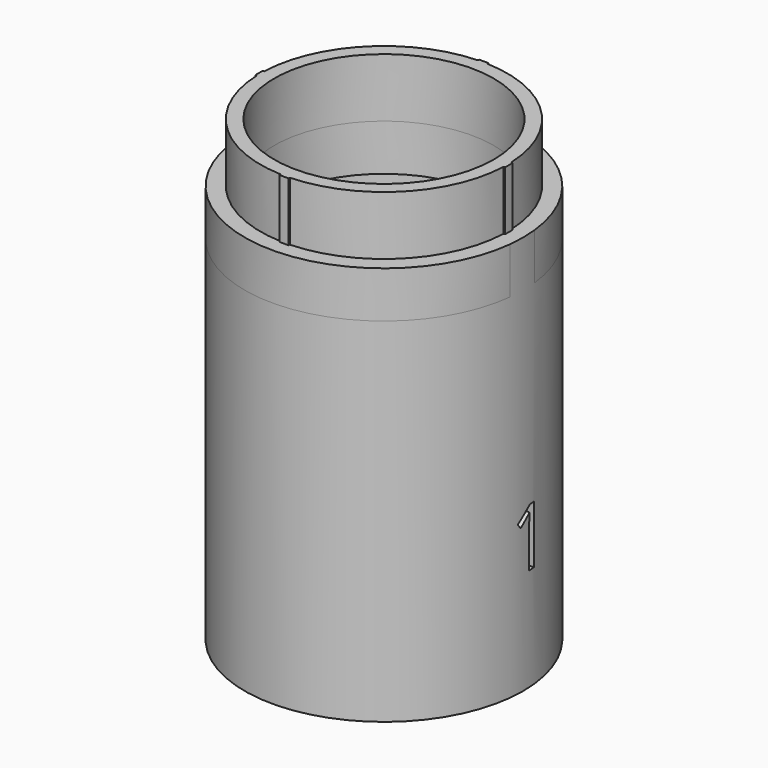
from build123d import *

# Parameters (mm, degrees)
F0_R         = 11.825
F1_DEPTH     = 6.35
F2_R         = 15
F2_R_2       = 13.45
F3_DEPTH     = 43
F4_R         = 15
F4_R_2       = 11.825
F5_DEPTH     = 5
F6_TEXT_SIZE = 8.7370552743
F7_DEPTH     = 25


# Not quite as in the source:
# - Text() gives the source's letters only with a copy of the font that has no kerning and outlines rounded to 1/6400 em; it was checked with that copy


with BuildPart() as f1:
    # F0 (on Top) → F1 (new body)
    with BuildSketch(Plane.XY):
        with BuildLine():
            ThreePointArc((13.2905981807, -0.5), (13.2976493374, -0.2500441932), (13.3, 0))
            ThreePointArc((13.3, 0), (13.2976493374, 0.2500441932), (13.2905981807, 0.5))
            ThreePointArc((13.2905981807, 0.5), (9.4045201898, 9.4045201898), (0.5, 13.2905981807))
            ThreePointArc((0.5, 13.2905981807), (0, 13.3), (-0.5, 13.2905981807))
            ThreePointArc((-0.5, 13.2905981807), (-9.4045201898, 9.4045201898), (-13.2905981807, 0.5))
            ThreePointArc((-13.2905981807, 0.5), (-13.3, 0), (-13.2905981807, -0.5))
            ThreePointArc((-13.2905981807, -0.5), (-9.4045201898, -9.4045201898), (-0.5, -13.2905981807))
            ThreePointArc((-0.5, -13.2905981807), (0, -13.3), (0.5, -13.2905981807))
            ThreePointArc((0.5, -13.2905981807), (9.4045201898, -9.4045201898), (13.2905981807, -0.5))
        make_face()
        Circle(F0_R, mode=Mode.SUBTRACT)
        with BuildLine():
            ThreePointArc((13.2905981807, 0.5), (13.2976493374, 0.2500441932), (13.3, 0))
            ThreePointArc((13.3, 0), (13.2976493374, -0.2500441932), (13.2905981807, -0.5))
            Line((13.2905981807, -0.5), (13.4407031066, -0.5))
            ThreePointArc((13.4407031066, -0.5), (13.45, 0), (13.4407031066, 0.5))
            Line((13.4407031066, 0.5), (13.2905981807, 0.5))
        make_face()
        with BuildLine():
            ThreePointArc((-0.5, 13.2905981807), (0, 13.3), (0.5, 13.2905981807))
            Line((0.5, 13.2905981807), (0.5, 13.4407031066))
            ThreePointArc((0.5, 13.4407031066), (0, 13.45), (-0.5, 13.4407031066))
            Line((-0.5, 13.4407031066), (-0.5, 13.2905981807))
        make_face()
        with BuildLine():
            Line((0.5, -13.4407031066), (0.5, -13.2905981807))
            ThreePointArc((0.5, -13.2905981807), (0, -13.3), (-0.5, -13.2905981807))
            Line((-0.5, -13.2905981807), (-0.5, -13.4407031066))
            ThreePointArc((-0.5, -13.4407031066), (0, -13.45), (0.5, -13.4407031066))
        make_face()
        with BuildLine():
            ThreePointArc((-13.2905981807, -0.5), (-13.3, 0), (-13.2905981807, 0.5))
            Line((-13.2905981807, 0.5), (-13.4407031066, 0.5))
            ThreePointArc((-13.4407031066, 0.5), (-13.45, 0), (-13.4407031066, -0.5))
            Line((-13.4407031066, -0.5), (-13.2905981807, -0.5))
        make_face()
    extrude(amount=F1_DEPTH)

    # F2 (on Top) → F3 (join)
    with BuildSketch(Plane.XY):
        Circle(F2_R)
        Circle(F2_R_2, mode=Mode.SUBTRACT)
    extrude(amount=-F3_DEPTH)

    # F6 (on Right) → F7 (cut)
    with BuildSketch(Plane.YZ):
        with Locations((-1.5248891784, -31.9193787873)):
            Text('1', F6_TEXT_SIZE, font='Open Sans', text_align=(TextAlign.LEFT, TextAlign.BOTTOM))
    extrude(amount=F7_DEPTH, mode=Mode.SUBTRACT)


with BuildPart() as f5:
    # F4 (on Top) → F5 (new body)
    with BuildSketch(Plane.XY):
        Circle(F4_R)
        Circle(F4_R_2, mode=Mode.SUBTRACT)
    extrude(amount=-F5_DEPTH)


solid = Compound([f1.part, f5.part])
